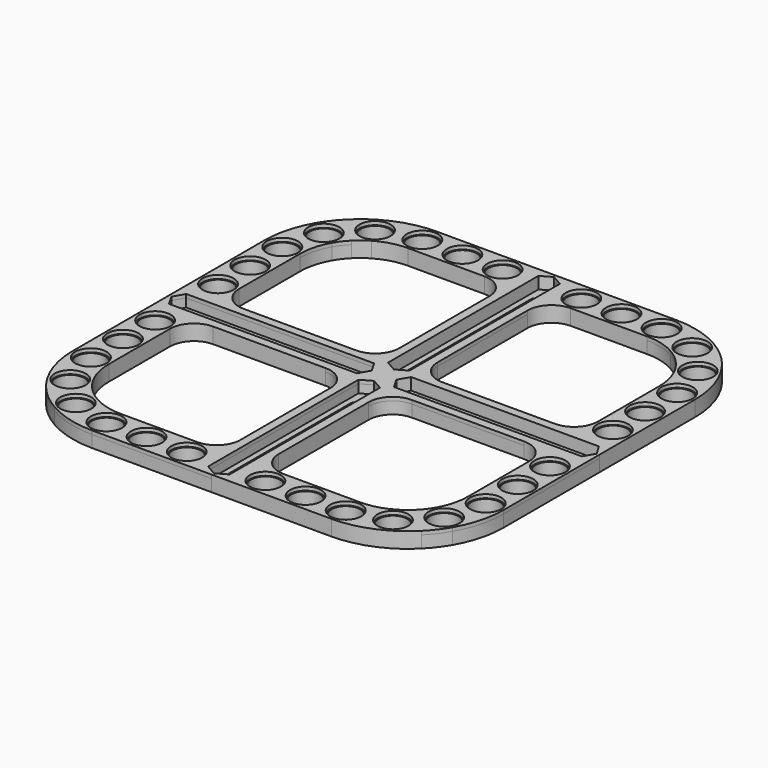
from build123d import *

# Parameters (mm, degrees)
F0_R     = 6.5
F0_R_2   = 6.5350000051
F0_R_3   = 6
F1_DEPTH = 5
F2_DEPTH = 3.5
F3_DEPTH = 1.5
F5_R     = 10
F6_COUNT = 4


# Not quite as in the source:
# - a feature names something its author has since deleted; it is built from what else it names


with BuildPart() as f1:
    # F0 (on Top) → F1 (new body)
    with BuildSketch(Plane.XY):
        with BuildLine():
            Line((5.5, -86.8245735195), (0, -90))
            Line((0, -90), (16.435, -90))
            ThreePointArc((16.435, -90), (8.935, -82.5), (16.435, -75))
            Line((16.435, -75), (8, -75))
            Line((8, -75), (8, -8.6188021535))
            Line((8, -8.6188021535), (5.5, -7.1754264805))
            Line((5.5, -7.1754264805), (5.5, -86.8245735195))
        make_face()
        with BuildLine():
            Line((5.5, -86.8245735195), (0, -90))
            Line((0, -90), (16.435, -90))
            ThreePointArc((16.435, -90), (8.935, -82.5), (16.435, -75))
            Line((16.435, -75), (8, -75))
            Line((8, -75), (8, -8.6188021535))
            Line((8, -8.6188021535), (5.5, -7.1754264805))
            Line((5.5, -7.1754264805), (5.5, -86.8245735195))
        make_face()
        with BuildLine():
            Line((0, -81.2458149392), (0, -88.8452994616))
            Line((0, -88.8452994616), (4.5, -86.2472232503))
            Line((4.5, -86.2472232503), (4.5, -7.7527767497))
            Line((4.5, -7.7527767497), (0, -5.1547005384))
            Line((0, -5.1547005384), (0, -12.7541850608))
            ThreePointArc((0, -12.7541850608), (1.4849242405, -13.3692608203), (2.1, -14.8541850608))
            Line((2.1, -14.8541850608), (2.1, -79.1458149392))
            ThreePointArc((2.1, -79.1458149392), (1.4849242405, -80.6307391797), (0, -81.2458149392))
        make_face()
        with BuildLine():
            ThreePointArc((33.235, -75), (25.735, -82.5), (33.235, -90))
            ThreePointArc((33.235, -90), (38.5383008589, -87.8033008589), (40.735, -82.5))
            ThreePointArc((40.735, -82.5), (38.5383008589, -77.1966991411), (33.235, -75))
        make_face()
        with Locations((33.235, -82.5)):
            Circle(F0_R, mode=Mode.SUBTRACT)
        with BuildLine():
            ThreePointArc((50, -75), (42.5, -82.5), (50, -90))
            ThreePointArc((50, -90), (55.3033008589, -87.8033008589), (57.5, -82.5))
            ThreePointArc((57.5, -82.5), (55.3033008589, -77.1966991411), (50, -75))
        make_face()
        with Locations((50, -82.5)):
            Circle(F0_R_2, mode=Mode.SUBTRACT)
        with BuildLine():
            ThreePointArc((62.5072897676, -71.6464247087), (59.7655489712, -81.8925390882), (70.0116634109, -84.6342796594))
            ThreePointArc((70.0116634109, -84.6342796594), (72.7552982665, -81.8892586249), (73.7594764465, -78.1403522665))
            ThreePointArc((73.7594764465, -78.1403522665), (70.0083829476, -71.644530529), (62.5072897676, -71.6464247087))
        make_face()
        with Locations((66.2594764465, -78.1403522665)):
            Circle(F0_R, mode=Mode.SUBTRACT)
        with BuildLine():
            ThreePointArc((16.435, -75), (8.935, -82.5), (16.435, -90))
            ThreePointArc((16.435, -90), (21.7383008589, -87.8033008589), (23.935, -82.5))
            ThreePointArc((23.935, -82.5), (21.7383008589, -77.1966991411), (16.435, -75))
        make_face()
        with Locations((16.435, -82.5)):
            Circle(F0_R, mode=Mode.SUBTRACT)
        with Locations((50, -82.5)):
            Circle(F0_R_2)
        with Locations((50.035, -82.4999811538)):
            Circle(F0_R_3, mode=Mode.SUBTRACT)
        with Locations((16.435, -82.5)):
            Circle(F0_R)
        with Locations((16.435, -82.5)):
            Circle(F0_R_3, mode=Mode.SUBTRACT)
        with Locations((33.235, -82.5)):
            Circle(F0_R)
        with Locations((33.235, -82.5)):
            Circle(F0_R_3, mode=Mode.SUBTRACT)
        with Locations((66.2594764465, -78.1403522665)):
            Circle(F0_R)
        with Locations((66.2594764465, -78.1403522665)):
            Circle(F0_R_3, mode=Mode.SUBTRACT)
        Polygon((0, -88.8452994616), (0, -90), (5.5, -86.8245735195), (5.5, -7.1754264805), (0, -4), (0, -5.1547005384), (4.5, -7.7527767497), (4.5, -86.2472232503), align=None)
        with BuildLine():
            ThreePointArc((57.5, -82.5), (55.3033008589, -87.8033008589), (50, -90))
            ThreePointArc((50, -90), (60.3592667121, -88.6352894798), (70.0116634109, -84.6342796594))
            ThreePointArc((70.0116634109, -84.6342796594), (59.7655489712, -81.8925390882), (62.5072897676, -71.6464247087))
            ThreePointArc((62.5072897676, -71.6464247087), (56.4745417707, -74.1470559046), (50, -75))
            ThreePointArc((50, -75), (55.3033008589, -77.1966991411), (57.5, -82.5))
        make_face()
        with BuildLine():
            ThreePointArc((23.935, -82.5), (21.7383008589, -87.8033008589), (16.435, -90))
            Line((16.435, -90), (33.235, -90))
            ThreePointArc((33.235, -90), (25.735, -82.5), (33.235, -75))
            Line((33.235, -75), (16.435, -75))
            ThreePointArc((16.435, -75), (21.7383008589, -77.1966991411), (23.935, -82.5))
        make_face()
        with BuildLine():
            ThreePointArc((40.735, -82.5), (38.5383008589, -87.8033008589), (33.235, -90))
            Line((33.235, -90), (50, -90))
            ThreePointArc((50, -90), (42.5, -82.5), (50, -75))
            Line((50, -75), (33.235, -75))
            ThreePointArc((33.235, -75), (38.5383008589, -77.1966991411), (40.735, -82.5))
        make_face()
        with BuildLine():
            ThreePointArc((73.7594764465, -78.1403522665), (72.7552982665, -81.8892586249), (70.0116634109, -84.6342796594))
            ThreePointArc((70.0116634109, -84.6342796594), (74.3557996756, -81.7300334409), (78.2842712475, -78.2842712475))
            Line((78.2842712475, -78.2842712475), (67.6776695297, -67.6776695297))
            ThreePointArc((67.6776695297, -67.6776695297), (65.2223748595, -69.8312708528), (62.5072897676, -71.6464247087))
            ThreePointArc((62.5072897676, -71.6464247087), (70.0083829476, -71.644530529), (73.7594764465, -78.1403522665))
        make_face()
        Polygon((0, -4), (5.5, -7.1754264805), (8, -8.6188021535), (8, -8), (0, 0), align=None)
        Polygon((0, -4), (5.5, -7.1754264805), (8, -8.6188021535), (8, -8), (0, 0), align=None)
    extrude(amount=-F1_DEPTH)

    # F0 (on Top) → F2 (cut)
    with BuildSketch(Plane.XY):
        with BuildLine():
            Line((0, -81.2458149392), (0, -88.8452994616))
            Line((0, -88.8452994616), (4.5, -86.2472232503))
            Line((4.5, -86.2472232503), (4.5, -7.7527767497))
            Line((4.5, -7.7527767497), (0, -5.1547005384))
            Line((0, -5.1547005384), (0, -12.7541850608))
            ThreePointArc((0, -12.7541850608), (1.4849242405, -13.3692608203), (2.1, -14.8541850608))
            Line((2.1, -14.8541850608), (2.1, -79.1458149392))
            ThreePointArc((2.1, -79.1458149392), (1.4849242405, -80.6307391797), (0, -81.2458149392))
        make_face()
    extrude(amount=-F2_DEPTH, mode=Mode.SUBTRACT)

    # F0 (on Top) → F3 (join)
    with BuildSketch(Plane.XY):
        with BuildLine():
            ThreePointArc((16.435, -75), (8.935, -82.5), (16.435, -90))
            ThreePointArc((16.435, -90), (21.7383008589, -87.8033008589), (23.935, -82.5))
            ThreePointArc((23.935, -82.5), (21.7383008589, -77.1966991411), (16.435, -75))
        make_face()
        with Locations((16.435, -82.5)):
            Circle(F0_R, mode=Mode.SUBTRACT)
        with BuildLine():
            ThreePointArc((33.235, -75), (25.735, -82.5), (33.235, -90))
            ThreePointArc((33.235, -90), (38.5383008589, -87.8033008589), (40.735, -82.5))
            ThreePointArc((40.735, -82.5), (38.5383008589, -77.1966991411), (33.235, -75))
        make_face()
        with Locations((33.235, -82.5)):
            Circle(F0_R, mode=Mode.SUBTRACT)
        with BuildLine():
            ThreePointArc((50, -75), (42.5, -82.5), (50, -90))
            ThreePointArc((50, -90), (55.3033008589, -87.8033008589), (57.5, -82.5))
            ThreePointArc((57.5, -82.5), (55.3033008589, -77.1966991411), (50, -75))
        make_face()
        with Locations((50, -82.5)):
            Circle(F0_R_2, mode=Mode.SUBTRACT)
        with BuildLine():
            ThreePointArc((62.5072897676, -71.6464247087), (59.7655489712, -81.8925390882), (70.0116634109, -84.6342796594))
            ThreePointArc((70.0116634109, -84.6342796594), (72.7552982665, -81.8892586249), (73.7594764465, -78.1403522665))
            ThreePointArc((73.7594764465, -78.1403522665), (70.0083829476, -71.644530529), (62.5072897676, -71.6464247087))
        make_face()
        with Locations((66.2594764465, -78.1403522665)):
            Circle(F0_R, mode=Mode.SUBTRACT)
        Polygon((0, -88.8452994616), (0, -90), (5.5, -86.8245735195), (5.5, -7.1754264805), (0, -4), (0, -5.1547005384), (4.5, -7.7527767497), (4.5, -86.2472232503), align=None)
        with BuildLine():
            Line((5.5, -86.8245735195), (0, -90))
            Line((0, -90), (16.435, -90))
            ThreePointArc((16.435, -90), (8.935, -82.5), (16.435, -75))
            Line((16.435, -75), (8, -75))
            Line((8, -75), (8, -8.6188021535))
            Line((8, -8.6188021535), (5.5, -7.1754264805))
            Line((5.5, -7.1754264805), (5.5, -86.8245735195))
        make_face()
        with BuildLine():
            ThreePointArc((23.935, -82.5), (21.7383008589, -87.8033008589), (16.435, -90))
            Line((16.435, -90), (33.235, -90))
            ThreePointArc((33.235, -90), (25.735, -82.5), (33.235, -75))
            Line((33.235, -75), (16.435, -75))
            ThreePointArc((16.435, -75), (21.7383008589, -77.1966991411), (23.935, -82.5))
        make_face()
        with BuildLine():
            ThreePointArc((40.735, -82.5), (38.5383008589, -87.8033008589), (33.235, -90))
            Line((33.235, -90), (50, -90))
            ThreePointArc((50, -90), (42.5, -82.5), (50, -75))
            Line((50, -75), (33.235, -75))
            ThreePointArc((33.235, -75), (38.5383008589, -77.1966991411), (40.735, -82.5))
        make_face()
        with BuildLine():
            ThreePointArc((57.5, -82.5), (55.3033008589, -87.8033008589), (50, -90))
            ThreePointArc((50, -90), (60.3592667121, -88.6352894798), (70.0116634109, -84.6342796594))
            ThreePointArc((70.0116634109, -84.6342796594), (59.7655489712, -81.8925390882), (62.5072897676, -71.6464247087))
            ThreePointArc((62.5072897676, -71.6464247087), (56.4745417707, -74.1470559046), (50, -75))
            ThreePointArc((50, -75), (55.3033008589, -77.1966991411), (57.5, -82.5))
        make_face()
        with BuildLine():
            ThreePointArc((73.7594764465, -78.1403522665), (72.7552982665, -81.8892586249), (70.0116634109, -84.6342796594))
            ThreePointArc((70.0116634109, -84.6342796594), (74.3557996756, -81.7300334409), (78.2842712475, -78.2842712475))
            Line((78.2842712475, -78.2842712475), (67.6776695297, -67.6776695297))
            ThreePointArc((67.6776695297, -67.6776695297), (65.2223748595, -69.8312708528), (62.5072897676, -71.6464247087))
            ThreePointArc((62.5072897676, -71.6464247087), (70.0083829476, -71.644530529), (73.7594764465, -78.1403522665))
        make_face()
        Polygon((0, -4), (5.5, -7.1754264805), (8, -8.6188021535), (8, -8), (0, 0), align=None)
        Polygon((0, -4), (5.5, -7.1754264805), (8, -8.6188021535), (8, -8), (0, 0), align=None)
    extrude(amount=F3_DEPTH)

    # F4: F1 across face


with BuildPart() as f1_1:
    add(f1.part)
    add(f1.part.mirror(Plane(origin=(4, -4, -1.75), x_dir=(-0.7071067812, 0.7071067812, 0), z_dir=(0.7071067812, 0.7071067812, 0))))

    # F5
    f5_edges = [f1_1.edges().sort_by_distance(p)[0] for p in [
        (8, -8, -1.75),
        (75, -8, -1.75),
        (8, -75, -1.75),
    ]]
    fillet(f5_edges, radius=F5_R)

    # F6: F1 ×4 about axis
    f6_axis = Axis((0, 0, -2.5), (0, 0, 1))


with BuildPart() as f1_2:
    add(f1_1.part)
    for i in range(1, F6_COUNT):
        add(f1_1.part.rotate(f6_axis, i * 360 / F6_COUNT))


solid = f1_2.part
